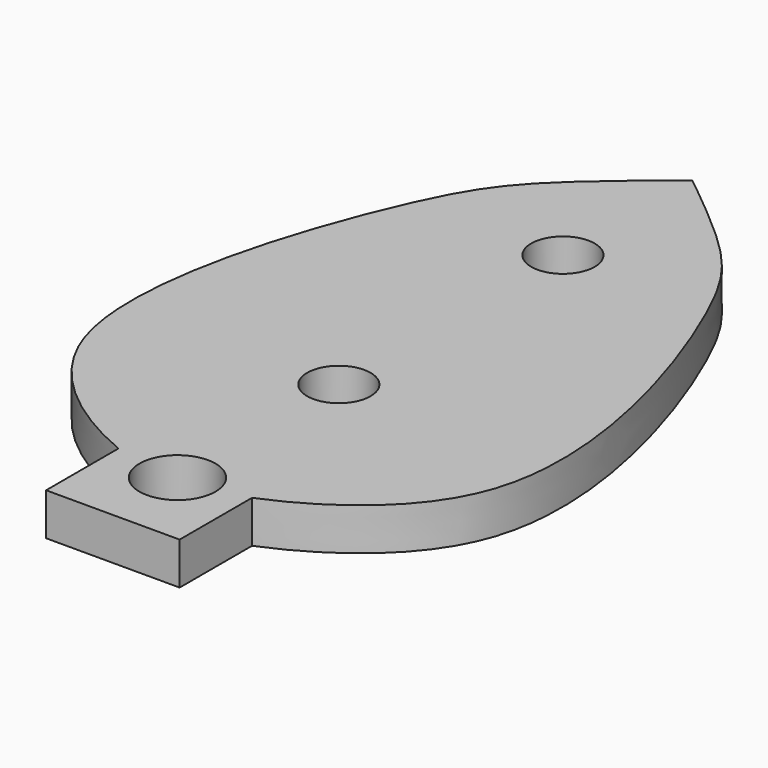
from build123d import *

# Parameters (mm, degrees)
F0_R     = 0.9
F0_R_2   = 0.75
F1_DEPTH = 1


with BuildPart() as f1:
    # F0 (on Top) → F1 (new body)
    with BuildSketch(Plane.XY):
        with BuildLine():
            Line((-1.5801185972, -14.1891559951), (0, -14.1891559951))
            Line((0, -14.1891559951), (1.5801185972, -14.1891559951))
            Line((1.5801185972, -14.1891559951), (1.5801185972, -12.0477042827))
            add(Edge.make_bspline(
                [(1.5801185972, -12.0477042827), (2.5459541843, -11.6559293479), (6.5291377224, -9.4358668754), (3.6630530699, -0.8044320957), (2.2592520144, 1.1687912571), (0.090530272, 2.877961005), (0.002861701, 2.946611466)],
                knots=[0, 0, 0, 0, 0.2531546654, 0.5920262082, 0.802833891, 0.9841362798, 0.9841362798, 0.9841362798, 0.9841362798], degree=3))
            add(Edge.make_bspline(
                [(0.002861701, 2.946611466), (0.0022873137, 2.9442752228), (0.0013231593, 2.9408383042), (0, 2.9359889357)],
                knots=[0.9959578645, 0.9959578645, 0.9959578645, 0.9959578645, 1, 1, 1, 1], degree=3))
            add(Edge.make_bspline(
                [(-0.002861701, 2.946611466), (-0.0022873137, 2.9442752228), (-0.0013231593, 2.9408383042), (0, 2.9359889357)],
                knots=[0.9959578645, 0.9959578645, 0.9959578645, 0.9959578645, 1, 1, 1, 1], degree=3))
            add(Edge.make_bspline(
                [(-1.5801185972, -12.0477042827), (-2.5459541843, -11.6559293479), (-6.5291377224, -9.4358668754), (-3.6630530699, -0.8044320957), (-2.2592520144, 1.1687912571), (-0.090530272, 2.877961005), (-0.002861701, 2.946611466)],
                knots=[0, 0, 0, 0, 0.2531546654, 0.5920262082, 0.802833891, 0.9841362798, 0.9841362798, 0.9841362798, 0.9841362798], degree=3))
            Line((-1.5801185972, -12.0477042827), (-1.5801185972, -14.1891559951))
        make_face()
        with Locations((0, -12.2777316719)):
            Circle(F0_R, mode=Mode.SUBTRACT)
        with Locations((0, -7.5046815909)):
            Circle(F0_R_2, mode=Mode.SUBTRACT)
        with Locations((0, -0.8759110351)):
            Circle(F0_R_2, mode=Mode.SUBTRACT)
        with BuildLine():
            add(Edge.make_bspline(
                [(0.002861701, 2.946611466), (0.0022873137, 2.9442752228), (0.0013231593, 2.9408383042), (0, 2.9359889357)],
                knots=[0.9959578645, 0.9959578645, 0.9959578645, 0.9959578645, 1, 1, 1, 1], degree=3))
            add(Edge.make_bspline(
                [(0.002861701, 2.946611466), (0.0017633731, 2.9474715315), (0.0008086746, 2.9482183335), (0, 2.9488501794)],
                knots=[0.9841362798, 0.9841362798, 0.9841362798, 0.9841362798, 0.9864076693, 0.9864076693, 0.9864076693, 0.9864076693], degree=3))
            add(Edge.make_bspline(
                [(-0.002861701, 2.946611466), (-0.0017633731, 2.9474715315), (-0.0008086746, 2.9482183335), (0, 2.9488501794)],
                knots=[0.9841362798, 0.9841362798, 0.9841362798, 0.9841362798, 0.9864076693, 0.9864076693, 0.9864076693, 0.9864076693], degree=3))
            add(Edge.make_bspline(
                [(-0.002861701, 2.946611466), (-0.0022873137, 2.9442752228), (-0.0013231593, 2.9408383042), (0, 2.9359889357)],
                knots=[0.9959578645, 0.9959578645, 0.9959578645, 0.9959578645, 1, 1, 1, 1], degree=3))
        make_face()
        with BuildLine():
            add(Edge.make_bspline(
                [(0.002861701, 2.946611466), (0.0017633731, 2.9474715315), (0.0008086746, 2.9482183335), (0, 2.9488501794)],
                knots=[0.9841362798, 0.9841362798, 0.9841362798, 0.9841362798, 0.9864076693, 0.9864076693, 0.9864076693, 0.9864076693], degree=3))
            add(Edge.make_bspline(
                [(0, 2.9488501794), (0.0034001215, 2.9515068139), (0.0042187835, 2.9521312164), (0.002861701, 2.946611466)],
                knots=[0.9864076693, 0.9864076693, 0.9864076693, 0.9864076693, 0.9959578645, 0.9959578645, 0.9959578645, 0.9959578645], degree=3))
        make_face()
        with BuildLine():
            add(Edge.make_bspline(
                [(0, 2.9488501794), (-0.0034001215, 2.9515068139), (-0.0042187835, 2.9521312164), (-0.002861701, 2.946611466)],
                knots=[0.9864076693, 0.9864076693, 0.9864076693, 0.9864076693, 0.9959578645, 0.9959578645, 0.9959578645, 0.9959578645], degree=3))
            add(Edge.make_bspline(
                [(-0.002861701, 2.946611466), (-0.0017633731, 2.9474715315), (-0.0008086746, 2.9482183335), (0, 2.9488501794)],
                knots=[0.9841362798, 0.9841362798, 0.9841362798, 0.9841362798, 0.9864076693, 0.9864076693, 0.9864076693, 0.9864076693], degree=3))
        make_face()
    extrude(amount=F1_DEPTH)


solid = f1.part
